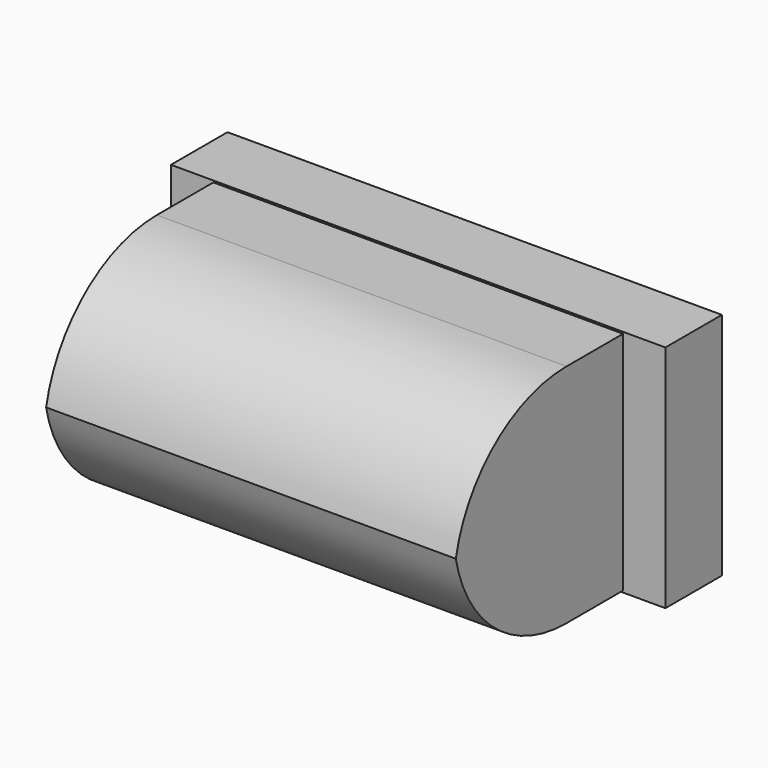
from build123d import *

# Parameters (mm, degrees)
F0_W        = 17.78
F0_H        = 8.255
F1_DEPTH    = 2.54
F2_W        = 14.732
F2_H        = 8.128
F3_DEPTH    = 10.16
F4_T1_DEPTH = 40.132


# Not quite as in the source:
# - a fillet or chamfer that OpenCascade refuses, or shapes differently, is made with other operations: its cross-section is extruded or revolved along the edge and cut away or added


with BuildPart() as f1:
    # F0 (on Front) → F1 (new body)
    with BuildSketch(Plane.XZ):
        Rectangle(F0_W, F0_H)
    extrude(amount=F1_DEPTH)

    # F2 (on Front) → F3 (join)
    with BuildSketch(Plane.XZ):
        Rectangle(F2_W, F2_H)
    extrude(amount=F3_DEPTH)

    # F4: fillet of radius 5.08 on 2 edges, made by hand

    # F4_s2 → F4_t1 (cut)
    with BuildSketch(Plane.YZ.offset(-20.066)):
        with BuildLine():
            ThreePointArc((-5.08, 4.064), (-8.6721024484, 2.5761024484), (-10.16, -1.016))
            Line((-10.16, -1.016), (-10.16, 4.064))
            Line((-10.16, 4.064), (-5.08, 4.064))
        make_face()
        with BuildLine():
            ThreePointArc((-5.08, -4.064), (-8.6721024484, -2.5761024484), (-10.16, 1.016))
            Line((-10.16, 1.016), (-10.16, -4.064))
            Line((-10.16, -4.064), (-5.08, -4.064))
        make_face()
    extrude(amount=F4_T1_DEPTH, mode=Mode.SUBTRACT)


solid = f1.part
